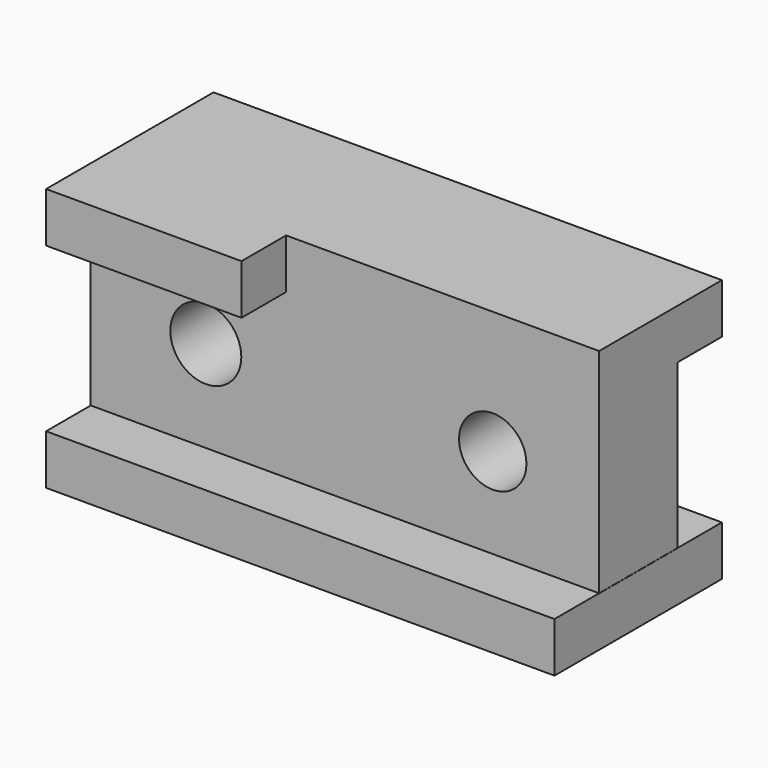
from build123d import *

# Parameters (mm, degrees)
F0_W          = 7.112
F0_H          = 6.35
F1_DEPTH      = 24.892
F3_DEPTH      = 64.77
F4_R          = 4.5216032169
F4_R_2        = 4.2905673548
F5_DEPTH      = 122.428
F5_DEPTH_BACK = 71.628


# Not quite as in the source:
# - a feature of the source that left no trace in its solid (it failed there, or was rolled back) is left out


with BuildPart() as f1:
    # F0 (on Right) → F1 (new body)
    with BuildSketch(Plane.YZ):
        with Locations((-8.5533469116, 0.5566177108)):
            Rectangle(F0_W, F0_H)
    extrude(amount=F1_DEPTH)

    # F0 (on Right) → F3 (join)
    with BuildSketch(Plane.YZ):
        with Locations((11.0046530884, 0.5566177108)):
            Rectangle(F0_W, F0_H)
        Polygon((7.4486530884, 3.7316177108), (-4.9973469116, 3.7316177108), (-4.9973469116, -2.6183822892), (-4.9973469116, -23.4382234705), (7.4486530884, -23.4382234705), (7.4486530884, -2.6183822892), align=None)
    extrude(amount=F3_DEPTH)

    # F4 (on Front) → F5 (cut, two sides)
    with BuildSketch(Plane.XZ) as f5_sk:
        with Locations((14.6613549441, -11.7537407205)):
            Circle(F4_R)
        with Locations((51.2163378298, -11.9365155697)):
            Circle(F4_R_2)
    extrude(amount=F5_DEPTH, mode=Mode.SUBTRACT)
    extrude(f5_sk.sketch, amount=-F5_DEPTH_BACK, mode=Mode.SUBTRACT)


with BuildPart() as f3:
    # F0 (on Right) → F3, piece 2 (new body)
    with BuildSketch(Plane.YZ):
        Polygon((-4.9973469116, -23.457913017), (-4.9973469116, -23.4382234705), (-12.1093469116, -23.4382234705), (-12.1093469116, -29.7882234705), (14.5606530884, -29.7882234705), (14.5606530884, -23.4382234705), (7.4486530884, -23.4382234705), (7.4486530884, -23.457913017), align=None)
    extrude(amount=F3_DEPTH)


solid = Compound([f1.part, f3.part])
